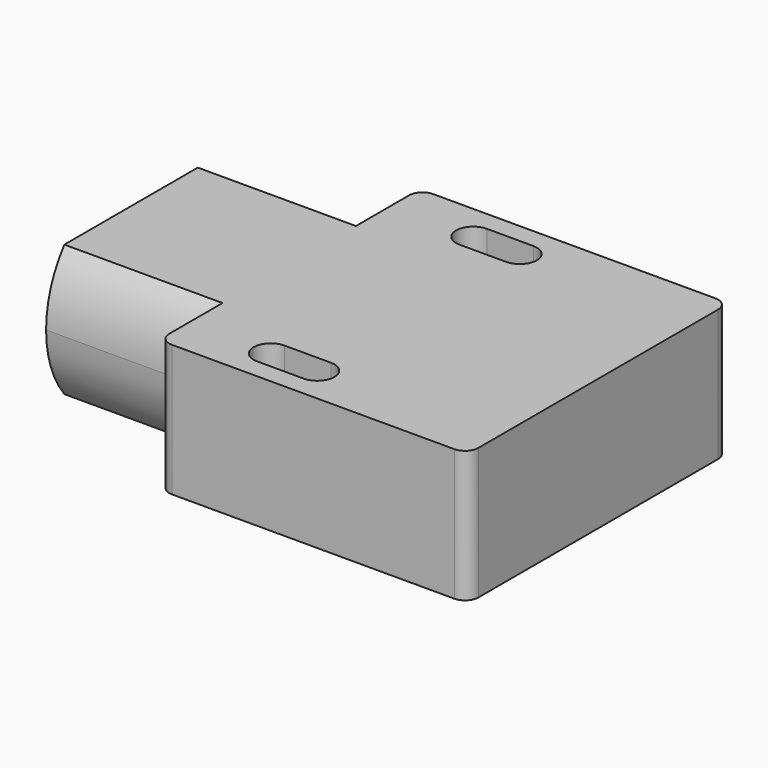
from build123d import *

# Parameters (mm, degrees)
F1_DEPTH = 12.4968
F3_R     = 1.27
F4_DEPTH = 15.0114


with BuildPart() as f1:
    # F0 (on Top) → F1 (new body)
    with BuildSketch(Plane.XY):
        Polygon((25.8765831087, -15.494), (25.8765831087, 15.494), (-3.4604168913, 15.494), (-3.4604168913, 10.0838), (-18.4718168913, 10.0838), (-18.4718168913, -10.0838), (-3.4604168913, -10.0838), (-3.4604168913, -15.494), align=None)
        with BuildLine():
            ThreePointArc((4.3881831087, -13.6271), (2.7625831087, -12.0015), (4.3881831087, -10.3759))
            Line((4.3881831087, -10.3759), (8.8077831087, -10.3759))
            ThreePointArc((8.8077831087, -10.3759), (10.4333831087, -12.0015), (8.8077831087, -13.6271))
            Line((8.8077831087, -13.6271), (4.3881831087, -13.6271))
        make_face(mode=Mode.SUBTRACT)
        with BuildLine():
            ThreePointArc((4.4008831087, 10.3759), (2.7752831087, 12.0015), (4.4008831087, 13.6271))
            Line((4.4008831087, 13.6271), (8.8204831087, 13.6271))
            ThreePointArc((8.8204831087, 13.6271), (10.4460831087, 12.0015), (8.8204831087, 10.3759))
            Line((8.8204831087, 10.3759), (4.4008831087, 10.3759))
        make_face(mode=Mode.SUBTRACT)
    extrude(amount=F1_DEPTH)

    # F3
    f3_edges = [f1.edges().sort_by_distance(p)[0] for p in [
        (-3.460417, -15.494, 6.2484),
        (-3.460417, 15.494, 6.2484),
        (25.876583, -15.494, 6.2484),
        (25.876583, 15.494, 6.2484),
    ]]
    fillet(f3_edges, radius=F3_R)

    # F2 (on face) → F4 (cut)
    with BuildSketch(Plane(origin=(-18.4718168913, 0, 0), x_dir=(0, -1, 0), z_dir=(-1, 0, 0))):
        with BuildLine():
            Line((10.0838, 0), (10.0838, 6.2484))
            ThreePointArc((10.0838, 6.2484), (9.5260702319, 2.9412851884), (7.9145764182, 0))
            Line((7.9145764182, 0), (10.0838, 0))
        make_face()
        with BuildLine():
            ThreePointArc((7.9145764182, 12.4968), (9.5260702319, 9.5555148116), (10.0838, 6.2484))
            Line((10.0838, 6.2484), (10.0838, 12.4968))
            Line((10.0838, 12.4968), (7.9145764182, 12.4968))
        make_face()
        with BuildLine():
            ThreePointArc((-7.9145764182, 0), (0, -3.8354), (7.9145764182, 0))
            Line((7.9145764182, 0), (-7.9145764182, 0))
        make_face()
        with BuildLine():
            ThreePointArc((-10.0838, 6.2484), (-9.5260702319, 9.5555148116), (-7.9145764182, 12.4968))
            Line((-7.9145764182, 12.4968), (-10.0838, 12.4968))
            Line((-10.0838, 12.4968), (-10.0838, 6.2484))
        make_face()
        with BuildLine():
            Line((-10.0838, 0), (-7.9145764182, 0))
            ThreePointArc((-7.9145764182, 0), (-9.5260702319, 2.9412851884), (-10.0838, 6.2484))
            Line((-10.0838, 6.2484), (-10.0838, 0))
        make_face()
    extrude(amount=-F4_DEPTH, mode=Mode.SUBTRACT)


solid = f1.part
